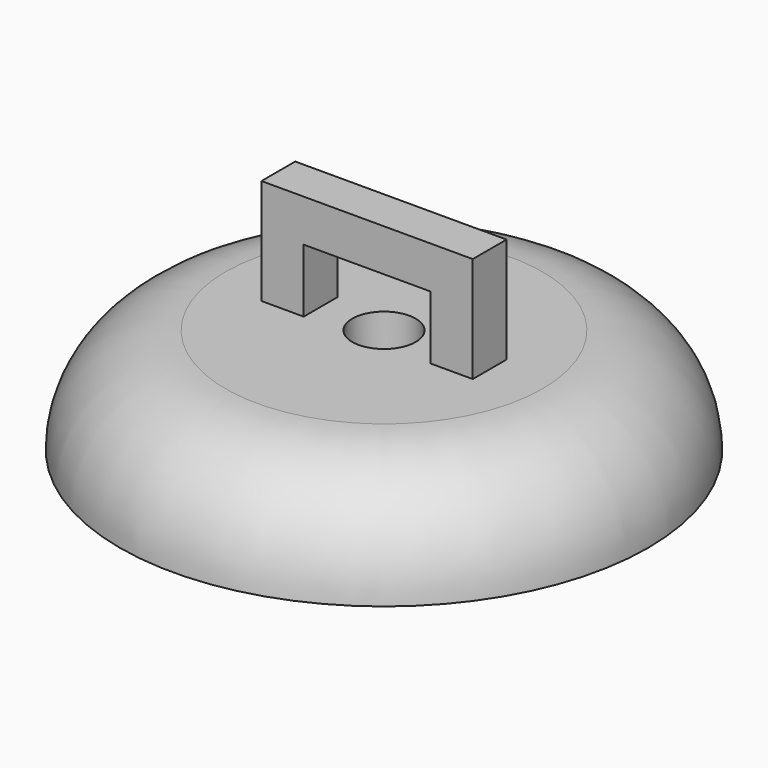
from build123d import *

# Parameters (mm, degrees)
F0_R     = 12.5
F1_DEPTH = 5
F2_R     = 4.99999
F3_T     = 2.5
F4_R     = 1.5
F5_DEPTH = 25
F6_W     = 2
F6_H     = 2
F7_DEPTH = 5
F8_W     = 2
F8_H     = 2
F9_DEPTH = 10


# Not quite as in the source:
# - a fillet or chamfer is up to 0.001 mm smaller than in the source, because OpenCascade refuses the exact size
# - a shell that OpenCascade refuses in one call is made with other operations: the cavity is built on its own and cut out


with BuildPart() as f1:
    # F0 (on Top) → F1 (new body)
    with BuildSketch(Plane.XY):
        Circle(F0_R)
    extrude(amount=F1_DEPTH)

    # F2 (radius 5 in the source; OpenCascade refuses exactly that, so slightly less here)
    f2_edges = [f1.edges().sort_by_distance(p)[0] for p in [
        (-12.5, 0, 5),
    ]]
    fillet(f2_edges, radius=F2_R)

    # F3: shell of thickness 2.5, made by hand


with BuildPart() as f3_core1:
    # F3_t2: copy of F1
    add(f1.part)

    # the walls: a layer under each face that stays
    f3_faces = [f3_core1.faces().sort_by_distance(p)[0] for p in [
        (-12.5, 0, 5e-06),
        (-11.0355368349, 0, 3.5355368349),
        (0, 0, 5),
    ]]
    thicken(f3_faces, amount=-F3_T, mode=Mode.SUBTRACT)


with BuildPart() as f1_1:
    add(f1.part)

    # what is left inside the walls is the cavity
    f3_cavity = [f3_core1.part.solids().sort_by_distance(p)[0] for p in [
        (0, -3.333333, 0.025),
    ]]
    add(f3_cavity, mode=Mode.SUBTRACT)

    # F4 (on face) → F5 (cut)
    with BuildSketch(Plane.XY.offset(5)):
        Circle(F4_R)
    extrude(amount=-F5_DEPTH, mode=Mode.SUBTRACT)

    # F6 (on face) → F7 (join)
    with BuildSketch(Plane.XY.offset(5)):
        with Locations((4, 0)):
            Rectangle(F6_W, F6_H)
        with Locations((-4, 0)):
            Rectangle(F6_W, F6_H)
    extrude(amount=F7_DEPTH)

    # F8 (on face) → F9 (join)
    with BuildSketch(Plane.YZ.offset(5)):
        with Locations((0, 9)):
            Rectangle(F8_W, F8_H)
    extrude(amount=-F9_DEPTH)


solid = f1_1.part
